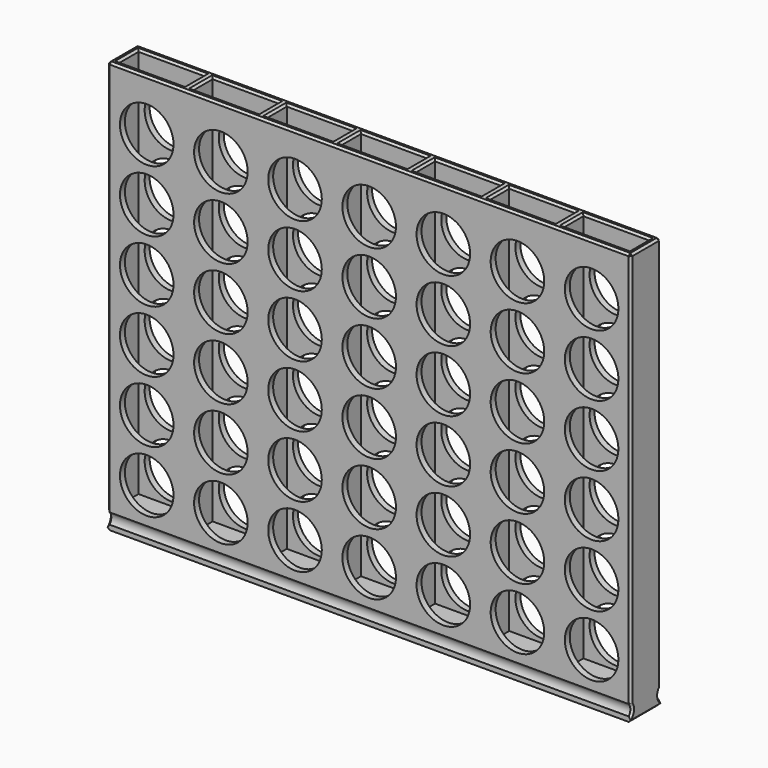
from build123d import *

# Parameters (mm, degrees)
F0_W     = 16
F0_H     = 6
F1_DEPTH = 95
F2_DEPTH = 5
F4_R     = 6.5
F5_DEPTH = 25
F6_DEPTH = 34.001
F7_R     = 2
F8_DEPTH = 127.001
F9_SIZE  = 0.49999


# Not quite as in the source:
# - a fillet or chamfer is up to 0.001 mm smaller than in the source, because OpenCascade refuses the exact size


with BuildPart() as f1:
    # F0 (on Top) → F1 (new body)
    with BuildSketch(Plane.XY):
        Polygon((-8, -4.5), (63.5, -4.5), (63.5, 4.5), (-26, 4.5), (-28, 4.5), (-44, 4.5), (-46, 4.5), (-63.5, 4.5), (-63.5, -4.5), (-28, -4.5), (-26, -4.5), (-10, -4.5), align=None)
        with Locations((-54, 0)):
            Rectangle(F0_W, F0_H, mode=Mode.SUBTRACT)
        with Locations((-36, 0)):
            Rectangle(F0_W, F0_H, mode=Mode.SUBTRACT)
        with Locations((-18, 0)):
            Rectangle(F0_W, F0_H, mode=Mode.SUBTRACT)
        Rectangle(F0_W, F0_H, mode=Mode.SUBTRACT)
        with Locations((18, 0)):
            Rectangle(F0_W, F0_H, mode=Mode.SUBTRACT)
        with Locations((36, 0)):
            Rectangle(F0_W, F0_H, mode=Mode.SUBTRACT)
        with Locations((54, 0)):
            Rectangle(F0_W, F0_H, mode=Mode.SUBTRACT)
    extrude(amount=F1_DEPTH)

    # F0 (on Top) → F2 (join)
    with BuildSketch(Plane.XY):
        Polygon((-8, -4.5), (63.5, -4.5), (63.5, 4.5), (-26, 4.5), (-28, 4.5), (-44, 4.5), (-46, 4.5), (-63.5, 4.5), (-63.5, -4.5), (-28, -4.5), (-26, -4.5), (-10, -4.5), align=None)
        with Locations((-54, 0)):
            Rectangle(F0_W, F0_H, mode=Mode.SUBTRACT)
        with Locations((-36, 0)):
            Rectangle(F0_W, F0_H, mode=Mode.SUBTRACT)
        with Locations((-18, 0)):
            Rectangle(F0_W, F0_H, mode=Mode.SUBTRACT)
        Rectangle(F0_W, F0_H, mode=Mode.SUBTRACT)
        with Locations((18, 0)):
            Rectangle(F0_W, F0_H, mode=Mode.SUBTRACT)
        with Locations((36, 0)):
            Rectangle(F0_W, F0_H, mode=Mode.SUBTRACT)
        with Locations((54, 0)):
            Rectangle(F0_W, F0_H, mode=Mode.SUBTRACT)
        with Locations((-54, 0)):
            Rectangle(F0_W, F0_H)
        with Locations((-36, 0)):
            Rectangle(F0_W, F0_H)
        with Locations((-18, 0)):
            Rectangle(F0_W, F0_H)
        Rectangle(F0_W, F0_H)
        with Locations((18, 0)):
            Rectangle(F0_W, F0_H)
        with Locations((36, 0)):
            Rectangle(F0_W, F0_H)
        with Locations((54, 0)):
            Rectangle(F0_W, F0_H)
    extrude(amount=-F2_DEPTH)

    # F4 (on face) → F5 (join)
    with BuildSketch(Plane.XZ.offset(4.5)):
        with Locations((-54, 82.5)):
            Circle(F4_R)
        with Locations((-54, 67.5)):
            Circle(F4_R)
        with Locations((-54, 52.5)):
            Circle(F4_R)
        with Locations((-54, 37.5)):
            Circle(F4_R)
        with Locations((-54, 22.5)):
            Circle(F4_R)
        with Locations((-54, 7.5)):
            Circle(F4_R)
        with Locations((54, 82.5)):
            Circle(F4_R)
        with Locations((54, 67.5)):
            Circle(F4_R)
        with Locations((54, 52.5)):
            Circle(F4_R)
        with Locations((54, 37.5)):
            Circle(F4_R)
        with Locations((54, 22.5)):
            Circle(F4_R)
        with Locations((54, 7.5)):
            Circle(F4_R)
        with Locations((18, 82.5)):
            Circle(F4_R)
        with Locations((18, 67.5)):
            Circle(F4_R)
        with Locations((18, 52.5)):
            Circle(F4_R)
        with Locations((18, 37.5)):
            Circle(F4_R)
        with Locations((18, 22.5)):
            Circle(F4_R)
        with Locations((18, 7.5)):
            Circle(F4_R)
        with Locations((-18, 82.5)):
            Circle(F4_R)
        with Locations((-18, 67.5)):
            Circle(F4_R)
        with Locations((-18, 52.5)):
            Circle(F4_R)
        with Locations((-18, 37.5)):
            Circle(F4_R)
        with Locations((-18, 22.5)):
            Circle(F4_R)
        with Locations((-18, 7.5)):
            Circle(F4_R)
        with Locations((-36, 82.5)):
            Circle(F4_R)
        with Locations((-36, 67.5)):
            Circle(F4_R)
        with Locations((-36, 52.5)):
            Circle(F4_R)
        with Locations((-36, 37.5)):
            Circle(F4_R)
        with Locations((-36, 22.5)):
            Circle(F4_R)
        with Locations((-36, 7.5)):
            Circle(F4_R)
        with Locations((0, 82.5)):
            Circle(F4_R)
        with Locations((0, 67.5)):
            Circle(F4_R)
        with Locations((0, 52.5)):
            Circle(F4_R)
        with Locations((0, 37.5)):
            Circle(F4_R)
        with Locations((0, 22.5)):
            Circle(F4_R)
        with Locations((0, 7.5)):
            Circle(F4_R)
        with Locations((36, 82.5)):
            Circle(F4_R)
        with Locations((36, 67.5)):
            Circle(F4_R)
        with Locations((36, 52.5)):
            Circle(F4_R)
        with Locations((36, 37.5)):
            Circle(F4_R)
        with Locations((36, 22.5)):
            Circle(F4_R)
        with Locations((36, 7.5)):
            Circle(F4_R)
    extrude(amount=F5_DEPTH)

    # F6 (cut, through all): faces of the model
    f6_faces = [f1.faces().sort_by_distance(p)[0] for p in [
        (-54, -29.5, 82.5),
        (-36, -29.5, 82.5),
        (-18, -29.5, 82.5),
        (0, -29.5, 82.5),
        (18, -29.5, 82.5),
        (36, -29.5, 82.5),
        (54, -29.5, 82.5),
        (54, -29.5, 67.5),
        (54, -29.5, 52.5),
        (54, -29.5, 37.5),
        (54, -29.5, 22.5),
        (54, -29.5, 7.5),
        (36, -29.5, 7.5),
        (36, -29.5, 22.5),
        (36, -29.5, 37.5),
        (36, -29.5, 52.5),
        (36, -29.5, 67.5),
        (18, -29.5, 67.5),
        (18, -29.5, 52.5),
        (18, -29.5, 37.5),
        (18, -29.5, 22.5),
        (18, -29.5, 7.5),
        (0, -29.5, 7.5),
        (0, -29.5, 22.5),
        (0, -29.5, 37.5),
        (0, -29.5, 52.5),
        (0, -29.5, 67.5),
        (-18, -29.5, 67.5),
        (-18, -29.5, 52.5),
        (-18, -29.5, 37.5),
        (-18, -29.5, 22.5),
        (-18, -29.5, 7.5),
        (-36, -29.5, 7.5),
        (-36, -29.5, 22.5),
        (-36, -29.5, 37.5),
        (-36, -29.5, 52.5),
        (-36, -29.5, 67.5),
        (-54, -29.5, 67.5),
        (-54, -29.5, 52.5),
        (-54, -29.5, 37.5),
        (-54, -29.5, 22.5),
        (-54, -29.5, 7.5),
    ]]
    extrude(f6_faces, amount=-F6_DEPTH, mode=Mode.SUBTRACT)

    # F7 (on face) → F8 (cut, through all)
    with BuildSketch(Plane(origin=(-63.5, 0, 0), x_dir=(0, -1, 0), z_dir=(-1, 0, 0))):
        with Locations((-6, -2.5)):
            Circle(F7_R)
        with Locations((6, -2.5)):
            Circle(F7_R)
    extrude(amount=-F8_DEPTH, mode=Mode.SUBTRACT)

    # F9 (size 0.5 in the source; OpenCascade refuses exactly that, so slightly less here)
    f9_edges = [f1.edges().sort_by_distance(p)[0] for p in [
        (-63.5, 4.5, 46.911438),
        (-63.5, -4.5, 46.911438),
        (0, 4.5, -5),
        (-63.5, 0, -5),
        (-63.5, 4, -2.5),
        (0, 4.5, 95),
        (-63.5, 0, 95),
        (0, -4.5, 95),
        (63.5, 0, 95),
        (63.5, 0, -5),
        (63.5, 4.5, 46.911438),
        (63.5, -4.5, 46.911438),
        (-63.5, -4, -2.5),
        (63.5, 4, -2.5),
        (63.5, -4, -2.5),
        (54, -3, 95),
        (46, 0, 95),
        (54, 3, 95),
        (62, 0, 95),
        (44, 0, 95),
        (36, 3, 95),
        (36, -3, 95),
        (8, 0, 95),
        (10, 0, 95),
        (18, 3, 95),
        (18, -3, 95),
        (26, 0, 95),
        (28, 0, 95),
        (0, 3, 95),
        (0, -3, 95),
        (-8, 0, 95),
        (-10, 0, 95),
        (-18, -3, 95),
        (-26, 0, 95),
        (-18, 3, 95),
        (-36, 3, 95),
        (-28, 0, 95),
        (-36, -3, 95),
        (-54, 3, 95),
        (-62, 0, 95),
        (-54, -3, 95),
        (-46, 0, 95),
        (-44, 0, 95),
    ]]
    chamfer(f9_edges, length=F9_SIZE)


solid = f1.part
